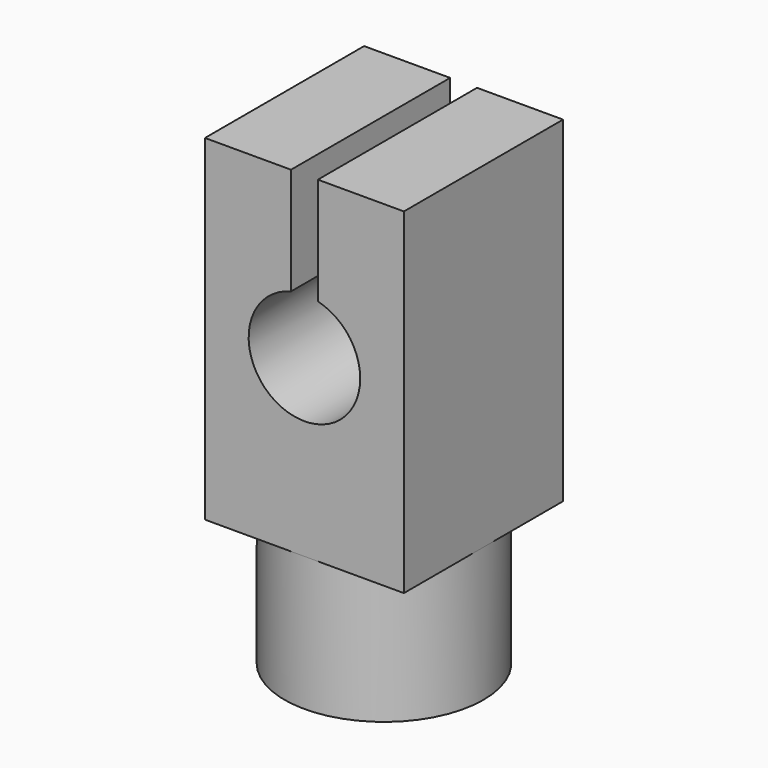
from build123d import *

# Parameters (mm, degrees)
F0_R     = 7.4
F1_DEPTH = 10
F2_W     = 14.8
F2_H     = 14.8
F3_DEPTH = 25
F5_DEPTH = 12.5


with BuildPart() as f1:
    # F0 (on Top) → F1 (new body)
    with BuildSketch(Plane.XY):
        Circle(F0_R)
    extrude(amount=-F1_DEPTH)

    # F2 (on face) → F3 (join)
    with BuildSketch(Plane.XY):
        Rectangle(F2_W, F2_H)
    extrude(amount=F3_DEPTH)

    # F4 (on Front) → F5 (cut, symmetric)
    with BuildSketch(Plane.XZ):
        with BuildLine():
            ThreePointArc((-1, 17.0277164746), (-2.5566090824, 9.7310169777), (4.15, 13))
            ThreePointArc((4.15, 13), (3.2689830223, 15.5566090824), (1, 17.0277164746))
            Line((1, 17.0277164746), (1, 13))
            Line((1, 13), (-1, 13))
            Line((-1, 13), (-1, 17.0277164746))
        make_face()
        with BuildLine():
            Line((1, 13), (1, 17.0277164746))
            ThreePointArc((1, 17.0277164746), (0, 17.15), (-1, 17.0277164746))
            Line((-1, 17.0277164746), (-1, 13))
            Line((-1, 13), (1, 13))
        make_face()
        with BuildLine():
            ThreePointArc((-1, 17.0277164746), (0, 17.15), (1, 17.0277164746))
            Line((1, 17.0277164746), (1, 25))
            Line((1, 25), (-1, 25))
            Line((-1, 25), (-1, 17.0277164746))
        make_face()
    extrude(amount=F5_DEPTH, both=True, mode=Mode.SUBTRACT)


solid = f1.part
